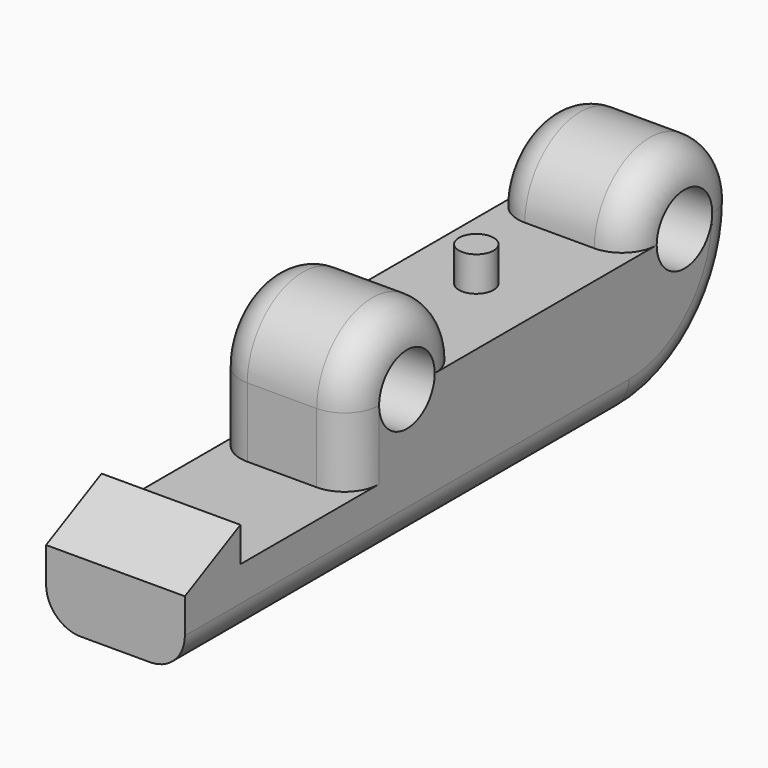
from build123d import *

# Parameters (mm, degrees)
F0_R     = 1.27
F1_DEPTH = 5.08
F2_R     = 0.635
F3_DEPTH = 1.27
F4_R     = 5.07999
F5_R     = 1.2699


# Not quite as in the source:
# - a fillet or chamfer is up to 0.001 mm smaller than in the source, because OpenCascade refuses the exact size


with BuildPart() as f1:
    # F0 (on Right) → F1 (new body)
    with BuildSketch(Plane.YZ):
        with BuildLine():
            ThreePointArc((-2.54, 0), (0, -2.54), (2.54, 0))
            ThreePointArc((2.54, 0), (0, 2.54), (-2.54, 0))
        make_face()
        Circle(F0_R, mode=Mode.SUBTRACT)
        with BuildLine():
            Line((10.16, 0), (2.54, 0))
            ThreePointArc((2.54, 0), (0, -2.54), (-2.54, 0))
            Line((-2.54, 0), (-2.54, -2.54))
            Line((-2.54, -2.54), (-2.54, -5.08))
            Line((-2.54, -5.08), (15.24, -5.08))
            Line((15.24, -5.08), (15.24, 0))
            ThreePointArc((15.24, 0), (12.7, -2.54), (10.16, 0))
        make_face()
        with BuildLine():
            ThreePointArc((15.24, 0), (12.7, 2.54), (10.16, 0))
            ThreePointArc((10.16, 0), (12.7, -2.54), (15.24, 0))
        make_face()
        with Locations((12.7, 0)):
            Circle(F0_R, mode=Mode.SUBTRACT)
        Polygon((-2.54, -5.08), (-2.54, -2.54), (-7.62, -2.54), (-10.16, -2.54), (-10.16, -5.08), align=None)
        Polygon((-10.16, -2.54), (-7.62, -2.54), (-7.62, -1.27), align=None)
    extrude(amount=F1_DEPTH)

    # F2 (on face) → F3 (join)
    with BuildSketch(Plane.XY):
        with Locations((2.54, 6.35)):
            Circle(F2_R)
    extrude(amount=F3_DEPTH)

    # F4 (radius 5.08 in the source; OpenCascade refuses exactly that, so slightly less here)
    f4_edges = [f1.edges().sort_by_distance(p)[0] for p in [
        (2.54, 15.24, -5.08),
    ]]
    fillet(f4_edges, radius=F4_R)

    # F5 (radius 1.27 in the source; OpenCascade refuses exactly that, so slightly less here)
    f5_edges = [f1.edges().sort_by_distance(p)[0] for p in [
        (5.08, 13.752105, -3.592105),
        (0, 13.752105, -3.592105),
        (5.08, 0, 2.54),
        (0, 0, 2.54),
    ]]
    fillet(f5_edges, radius=F5_R)


solid = f1.part
